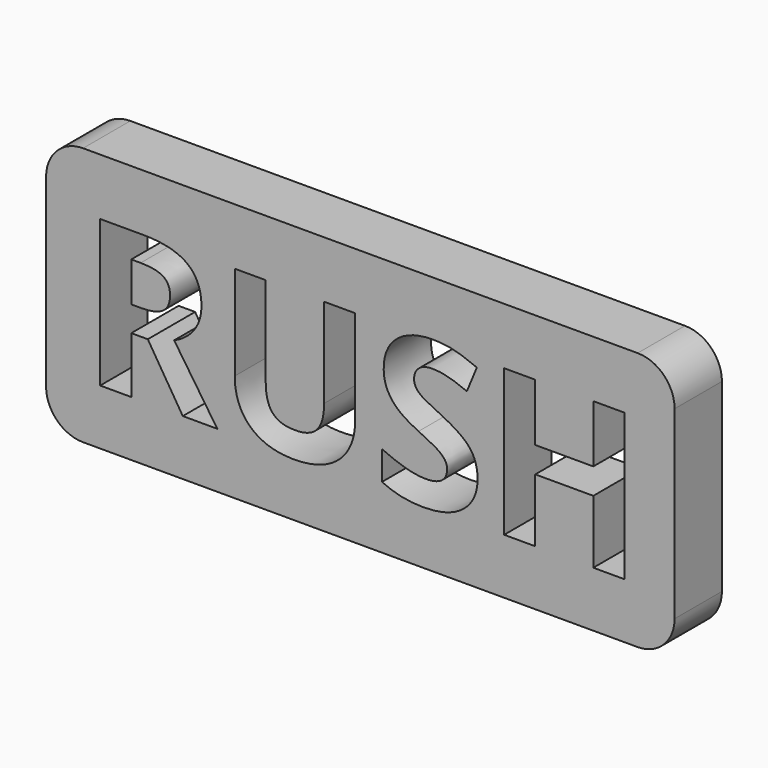
from build123d import *

# Parameters (mm, degrees)
F1_DEPTH     = 8
F2_TEXT_SIZE = 27.7777777778
F3_DEPTH     = 25


# Not quite as in the source:
# - Text() gives the source's letters only with a copy of the font that has no kerning and outlines rounded to 1/6400 em; it was checked with that copy


with BuildPart() as f1:
    # F0 (on Front) → F1 (new body)
    with BuildSketch(Plane.XZ):
        with BuildLine():
            Line((80, 0), (5, 0))
            ThreePointArc((5, 0), (1.4644660941, -1.4644660941), (0, -5))
            Line((0, -5), (0, -30))
            ThreePointArc((0, -30), (1.4644660941, -33.5355339059), (5, -35))
            Line((5, -35), (80, -35))
            ThreePointArc((80, -35), (83.5355339059, -33.5355339059), (85, -30))
            Line((85, -30), (85, -5))
            ThreePointArc((85, -5), (83.5355339059, -1.4644660941), (80, 0))
        make_face()
    extrude(amount=F1_DEPTH)

    # F2 (on face) → F3 (cut)
    with BuildSketch(Plane.XZ.offset(8)):
        with Locations((4.8177083333, -27.5)):
            Text('RUSH', F2_TEXT_SIZE, font='Open Sans', font_style=FontStyle.BOLD, text_align=(TextAlign.LEFT, TextAlign.BOTTOM))
    extrude(amount=-F3_DEPTH, mode=Mode.SUBTRACT)


solid = f1.part
